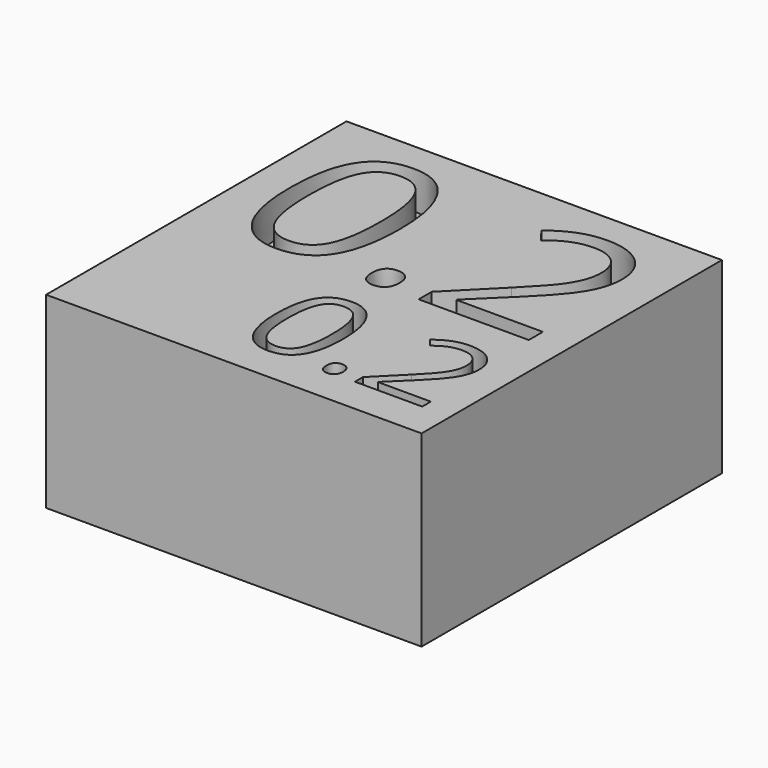
from build123d import *

# Parameters (mm, degrees)
F0_W           = 10
F0_H           = 10
F1_DEPTH       = 5
F2_TEXT_SIZE   = 6.25
F2_TEXT_SIZE_2 = 3.8194444444
F3_DEPTH       = 1


# Not quite as in the source:
# - a feature names something its author has since deleted; it is built from what else it names
# - Text() gives the source's letters only with a copy of the font that has no kerning and outlines rounded to 1/6400 em; it was checked with that copy


with BuildPart() as f1:
    # F0 (on Top) → F1 (new body)
    with BuildSketch(Plane.XY):
        Rectangle(F0_W, F0_H)
    extrude(amount=F1_DEPTH)

    # F2 (on face) → F3 (cut)
    with BuildSketch(Plane.XY.offset(5)):
        with Locations((-4.3617928759, -0.3220916566)):
            Text('0.2', F2_TEXT_SIZE, font='Open Sans', text_align=(TextAlign.LEFT, TextAlign.BOTTOM))
        with Locations((-0.9228301036, -4.0478505921)):
            Text('0.2', F2_TEXT_SIZE_2, font='Open Sans', text_align=(TextAlign.LEFT, TextAlign.BOTTOM))
    extrude(amount=-F3_DEPTH, mode=Mode.SUBTRACT)


solid = f1.part
